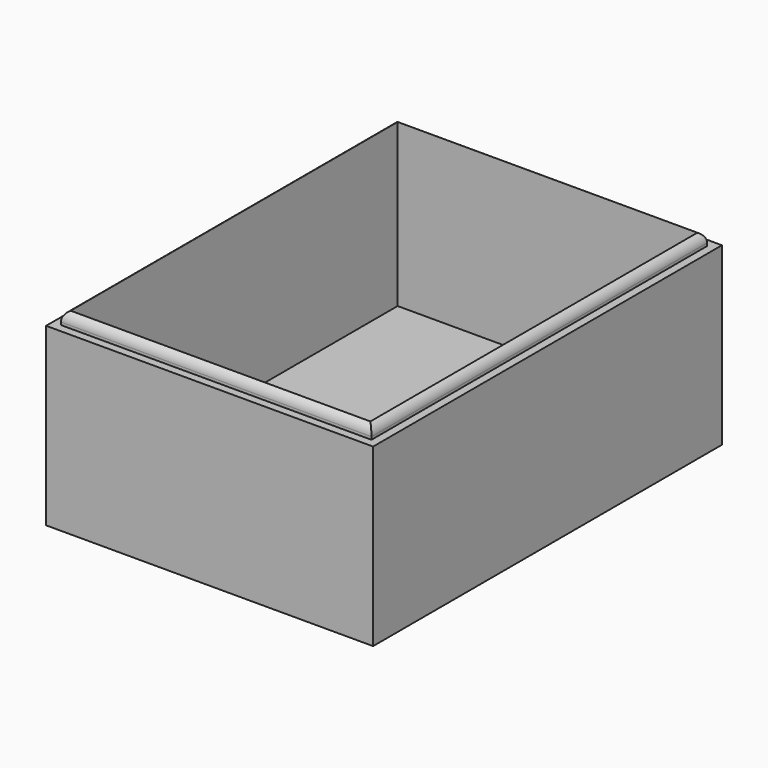
from build123d import *

# Parameters (mm, degrees)
F0_W         = 76.2
F0_H         = 101.6
F1_DEPTH     = 38.1
F2_W         = 69.85
F2_H         = 95.25
F3_DEPTH     = 34.925
F4_W         = 72.39
F4_H         = 97.79
F4_W_2       = 69.85
F4_H_2       = 95.25
F5_DEPTH     = 3.175
F6_W         = 76.2
F6_H         = 101.6
F6_W_2       = 73.66
F6_H_2       = 99.06
F7_DEPTH     = 3.175
F8_T1_DEPTH  = 110.49
F8_T3_DEPTH  = 85.09
F8_T5_DEPTH  = 99.06
F8_T7_DEPTH  = 73.66
F8_T13_DEPTH = 105.41
F8_T19_DEPTH = 80.01
F8_T28_DEPTH = 105.41
F8_T34_DEPTH = 80.01
F8_T43_DEPTH = 80.01
F8_T49_DEPTH = 105.41
F8_T58_DEPTH = 105.41
F8_T64_DEPTH = 80.01


# Not quite as in the source:
# - a fillet or chamfer that OpenCascade refuses, or shapes differently, is made with other operations: its cross-section is extruded or revolved along the edge and cut away or added


with BuildPart() as f1:
    # F0 (on Top) → F1 (new body)
    with BuildSketch(Plane.XY):
        Rectangle(F0_W, F0_H)
    extrude(amount=F1_DEPTH)

    # F2 (on face) → F3 (cut)
    with BuildSketch(Plane.XY.offset(38.1)):
        Rectangle(F2_W, F2_H)
    extrude(amount=-F3_DEPTH, mode=Mode.SUBTRACT)

    # F4 (on face) → F5 (join)
    with BuildSketch(Plane.XY.offset(38.1)):
        Rectangle(F4_W, F4_H)
        Rectangle(F4_W_2, F4_H_2, mode=Mode.SUBTRACT)
    extrude(amount=F5_DEPTH)

    # F6 (on face) → F7 (join)
    with BuildSketch(Plane(origin=(0, 0, 0), x_dir=(1, 0, 0), z_dir=(0, 0, -1))):
        Rectangle(F6_W, F6_H)
        Rectangle(F6_W_2, F6_H_2, mode=Mode.SUBTRACT)
    extrude(amount=F7_DEPTH)

    # F8: fillet of radius 2.54 on 8 edges, made by hand

    # F8_s2 → F8_t1 (cut)
    with BuildSketch(Plane.XZ.offset(-55.245)):
        with BuildLine():
            ThreePointArc((-33.655, 41.275), (-35.4510512242, 40.5310512242), (-36.195, 38.735))
            Line((-36.195, 38.735), (-36.195, 41.275))
            Line((-36.195, 41.275), (-33.655, 41.275))
        make_face()
        with BuildLine():
            ThreePointArc((36.195, 38.735), (35.4510512242, 40.5310512242), (33.655, 41.275))
            Line((33.655, 41.275), (36.195, 41.275))
            Line((36.195, 41.275), (36.195, 38.735))
        make_face()
    extrude(amount=F8_T1_DEPTH, mode=Mode.SUBTRACT)

    # F8_s4 → F8_t3 (cut)
    with BuildSketch(Plane.YZ.offset(-42.545)):
        with BuildLine():
            ThreePointArc((-46.355, 41.275), (-48.1510512242, 40.5310512242), (-48.895, 38.735))
            Line((-48.895, 38.735), (-48.895, 41.275))
            Line((-48.895, 41.275), (-46.355, 41.275))
        make_face()
        with BuildLine():
            ThreePointArc((46.355, 41.275), (48.1510512242, 40.5310512242), (48.895, 38.735))
            Line((48.895, 38.735), (48.895, 41.275))
            Line((48.895, 41.275), (46.355, 41.275))
        make_face()
    extrude(amount=F8_T3_DEPTH, mode=Mode.SUBTRACT)

    # F8_s6 → F8_t5 (cut)
    with BuildSketch(Plane.XZ.offset(-49.53)):
        with BuildLine():
            ThreePointArc((-39.37, -3.175), (-37.5739487758, -2.4310512242), (-36.83, -0.635))
            Line((-36.83, -0.635), (-36.83, -3.175))
            Line((-36.83, -3.175), (-39.37, -3.175))
        make_face()
        with BuildLine():
            ThreePointArc((39.37, -3.175), (37.5739487758, -2.4310512242), (36.83, -0.635))
            Line((36.83, -0.635), (36.83, -3.175))
            Line((36.83, -3.175), (39.37, -3.175))
        make_face()
    extrude(amount=F8_T5_DEPTH, mode=Mode.SUBTRACT)

    # F8_s8 → F8_t7 (cut)
    with BuildSketch(Plane.YZ.offset(-36.83)):
        with BuildLine():
            ThreePointArc((-52.07, -3.175), (-50.2739487758, -2.4310512242), (-49.53, -0.635))
            Line((-49.53, -0.635), (-49.53, -3.175))
            Line((-49.53, -3.175), (-52.07, -3.175))
        make_face()
        with BuildLine():
            ThreePointArc((52.07, -3.175), (50.2739487758, -2.4310512242), (49.53, -0.635))
            Line((49.53, -0.635), (49.53, -3.175))
            Line((49.53, -3.175), (52.07, -3.175))
        make_face()
    extrude(amount=F8_T7_DEPTH, mode=Mode.SUBTRACT)


with BuildPart() as f8_tool11:
    # F8_s12 → F8_t13 (new body)
    with BuildSketch(Plane.XZ.offset(-55.88)):
        with BuildLine():
            ThreePointArc((-39.37, -3.175), (-37.5739487758, -2.4310512242), (-36.83, -0.635))
            Line((-36.83, -0.635), (-36.83, -3.175))
            Line((-36.83, -3.175), (-39.37, -3.175))
        make_face()
    extrude(amount=F8_T13_DEPTH)

    split(bisect_by=Plane.XZ.offset(-49.53), keep=Keep.BOTTOM)

    split(bisect_by=Plane.YZ.offset(-38.1), keep=Keep.TOP)

    split(bisect_by=Plane.XZ.offset(-50.8), keep=Keep.TOP)


with BuildPart() as f8_tool17:
    # F8_s18 → F8_t19 (new body)
    with BuildSketch(Plane.YZ.offset(36.83)):
        with BuildLine():
            ThreePointArc((52.07, -3.175), (50.2739487758, -2.4310512242), (49.53, -0.635))
            Line((49.53, -0.635), (49.53, -3.175))
            Line((49.53, -3.175), (52.07, -3.175))
        make_face()
    extrude(amount=-F8_T19_DEPTH)

    split(bisect_by=Plane.YZ.offset(-36.83), keep=Keep.BOTTOM)

    split(bisect_by=Plane.YZ.offset(-38.1), keep=Keep.TOP)

    split(bisect_by=Plane.XZ.offset(-50.8), keep=Keep.TOP)


with BuildPart() as f8_tool11_1:
    add(f8_tool11.part)

    # F8_t23: intersect F8_tool17
    add(f8_tool17.part, mode=Mode.INTERSECT)


with BuildPart() as f1_1:
    add(f1.part)

    # F8_t9: cut F8_tool11
    add(f8_tool11_1.part, mode=Mode.SUBTRACT)


with BuildPart() as f8_tool26:
    # F8_s27 → F8_t28 (new body)
    with BuildSketch(Plane.XZ.offset(-49.53)):
        with BuildLine():
            ThreePointArc((-39.37, -3.175), (-37.5739487758, -2.4310512242), (-36.83, -0.635))
            Line((-36.83, -0.635), (-36.83, -3.175))
            Line((-36.83, -3.175), (-39.37, -3.175))
        make_face()
    extrude(amount=F8_T28_DEPTH)

    split(bisect_by=Plane.XZ.offset(49.53), keep=Keep.TOP)

    split(bisect_by=Plane.YZ.offset(-38.1), keep=Keep.TOP)

    split(bisect_by=Plane.XZ.offset(50.8), keep=Keep.BOTTOM)


with BuildPart() as f8_tool32:
    # F8_s33 → F8_t34 (new body)
    with BuildSketch(Plane.YZ.offset(-43.18)):
        with BuildLine():
            ThreePointArc((-52.07, -3.175), (-50.2739487758, -2.4310512242), (-49.53, -0.635))
            Line((-49.53, -0.635), (-49.53, -3.175))
            Line((-49.53, -3.175), (-52.07, -3.175))
        make_face()
    extrude(amount=F8_T34_DEPTH)

    split(bisect_by=Plane.YZ.offset(-36.83), keep=Keep.BOTTOM)

    split(bisect_by=Plane.YZ.offset(-38.1), keep=Keep.TOP)

    split(bisect_by=Plane.XZ.offset(50.8), keep=Keep.BOTTOM)


with BuildPart() as f8_tool26_1:
    add(f8_tool26.part)

    # F8_t38: intersect F8_tool32
    add(f8_tool32.part, mode=Mode.INTERSECT)


with BuildPart() as f1_2:
    add(f1_1.part)

    # F8_t24: cut F8_tool26
    add(f8_tool26_1.part, mode=Mode.SUBTRACT)


with BuildPart() as f8_tool41:
    # F8_s42 → F8_t43 (new body)
    with BuildSketch(Plane.YZ.offset(-36.83)):
        with BuildLine():
            ThreePointArc((-52.07, -3.175), (-50.2739487758, -2.4310512242), (-49.53, -0.635))
            Line((-49.53, -0.635), (-49.53, -3.175))
            Line((-49.53, -3.175), (-52.07, -3.175))
        make_face()
    extrude(amount=F8_T43_DEPTH)

    split(bisect_by=Plane.YZ.offset(38.1), keep=Keep.BOTTOM)

    split(bisect_by=Plane.YZ.offset(36.83), keep=Keep.TOP)

    split(bisect_by=Plane.XZ.offset(50.8), keep=Keep.BOTTOM)


with BuildPart() as f8_tool47:
    # F8_s48 → F8_t49 (new body)
    with BuildSketch(Plane.XZ.offset(55.88)):
        with BuildLine():
            ThreePointArc((39.37, -3.175), (37.5739487758, -2.4310512242), (36.83, -0.635))
            Line((36.83, -0.635), (36.83, -3.175))
            Line((36.83, -3.175), (39.37, -3.175))
        make_face()
    extrude(amount=-F8_T49_DEPTH)

    split(bisect_by=Plane.YZ.offset(38.1), keep=Keep.BOTTOM)

    split(bisect_by=Plane.XZ.offset(49.53), keep=Keep.TOP)

    split(bisect_by=Plane.XZ.offset(50.8), keep=Keep.BOTTOM)


with BuildPart() as f8_tool41_1:
    add(f8_tool41.part)

    # F8_t53: intersect F8_tool47
    add(f8_tool47.part, mode=Mode.INTERSECT)


with BuildPart() as f1_3:
    add(f1_2.part)

    # F8_t39: cut F8_tool41
    add(f8_tool41_1.part, mode=Mode.SUBTRACT)


with BuildPart() as f8_tool56:
    # F8_s57 → F8_t58 (new body)
    with BuildSketch(Plane.XZ.offset(49.53)):
        with BuildLine():
            ThreePointArc((39.37, -3.175), (37.5739487758, -2.4310512242), (36.83, -0.635))
            Line((36.83, -0.635), (36.83, -3.175))
            Line((36.83, -3.175), (39.37, -3.175))
        make_face()
    extrude(amount=-F8_T58_DEPTH)

    split(bisect_by=Plane.YZ.offset(38.1), keep=Keep.BOTTOM)

    split(bisect_by=Plane.XZ.offset(-49.53), keep=Keep.BOTTOM)

    split(bisect_by=Plane.XZ.offset(-50.8), keep=Keep.TOP)


with BuildPart() as f8_tool62:
    # F8_s63 → F8_t64 (new body)
    with BuildSketch(Plane.YZ.offset(43.18)):
        with BuildLine():
            ThreePointArc((52.07, -3.175), (50.2739487758, -2.4310512242), (49.53, -0.635))
            Line((49.53, -0.635), (49.53, -3.175))
            Line((49.53, -3.175), (52.07, -3.175))
        make_face()
    extrude(amount=-F8_T64_DEPTH)

    split(bisect_by=Plane.YZ.offset(38.1), keep=Keep.BOTTOM)

    split(bisect_by=Plane.YZ.offset(36.83), keep=Keep.TOP)

    split(bisect_by=Plane.XZ.offset(-50.8), keep=Keep.TOP)


with BuildPart() as f8_tool56_1:
    add(f8_tool56.part)

    # F8_t68: intersect F8_tool62
    add(f8_tool62.part, mode=Mode.INTERSECT)


with BuildPart() as f1_4:
    add(f1_3.part)

    # F8_t54: cut F8_tool56
    add(f8_tool56_1.part, mode=Mode.SUBTRACT)


solid = f1_4.part
